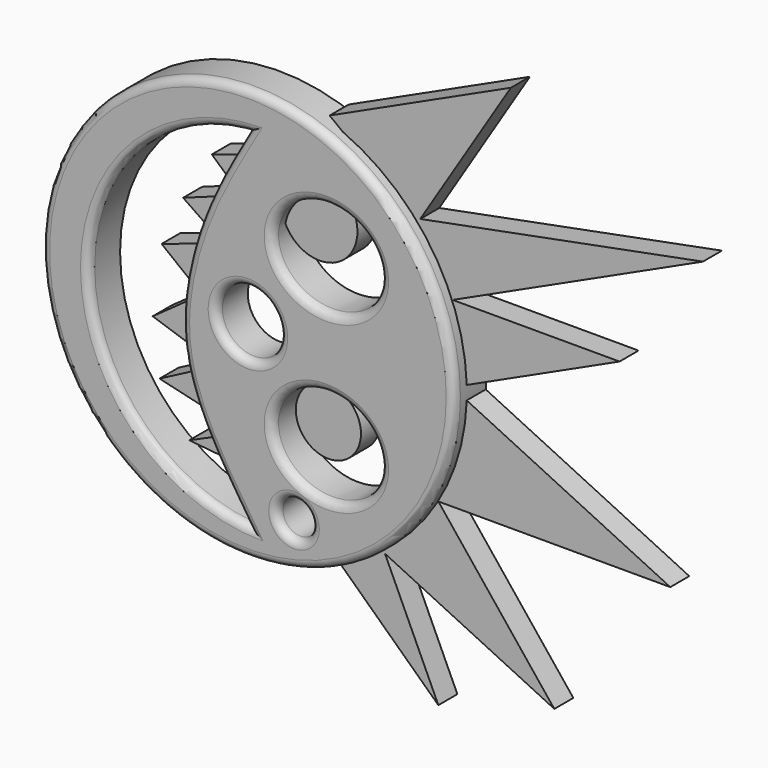
from build123d import *

# Parameters (mm, degrees)
F0_R     = 26.0210777057
F1_DEPTH = 5
F2_R     = 4.0159467608
F2_R_2   = 2.1900892751
F3_DEPTH = 5.0038
F4_R     = 4.7816675569
F5_DEPTH = 3
F4_R_2   = 4.1098377278
F6_R     = 1


# Not quite as in the source:
# - a feature names something its author has since deleted; it is built from what else it names


with BuildPart() as f1:
    # F0 (on Front) → F1 (new body)
    with BuildSketch(Plane.XZ):
        Circle(F0_R)
    extrude(amount=F1_DEPTH)

    # F2 (on face) → F3 (cut)
    with BuildSketch(Plane(origin=(0, 0, 0), x_dir=(-1, 0, 0), z_dir=(0, 1, 0))):
        with BuildLine():
            add(Edge.make_bspline(
                [(-3.0610915273, 10.4437181726), (-3.0610915273, 20.7679885804), (-13.3247473277, 15.6058533765), (-23.5884031281, 10.4437181726), (-13.3247473277, 5.2815829687), (-3.0610915273, 0.1194477649), (-3.0610915273, 10.4437181726)],
                knots=[0, 0, 0, 2.0943951024, 2.0943951024, 4.1887902048, 4.1887902048, 6.2831853072, 6.2831853072, 6.2831853072], degree=2, weights=[1, 0.5, 1, 0.5, 1, 0.5, 1]))
        make_face()
        with BuildLine():
            add(Edge.make_bspline(
                [(-3.0610915273, -10.4437181726), (-3.0610915273, -0.1194477649), (-13.3247473277, -5.2815829687), (-23.5884031281, -10.4437181726), (-13.3247473277, -15.6058533765), (-3.0610915273, -20.7679885804), (-3.0610915273, -10.4437181726)],
                knots=[0, 0, 0, 2.0943951024, 2.0943951024, 4.1887902048, 4.1887902048, 6.2831853072, 6.2831853072, 6.2831853072], degree=2, weights=[1, 0.5, 1, 0.5, 1, 0.5, 1]))
        make_face()
        with BuildLine():
            add(Edge.make_bspline(
                [(0, 21.2571714073), (2.1395691334, 17.5349161848), (6.4343134883, 10.0632554868), (9.437117435, -3.3422966836), (5.9538411419, -13.4085659123), (2.0003803602, -19.410914793), (0, -22.4479958415)],
                knots=[0, 0, 0, 0, 0.2628002315, 0.5275173365, 0.7609322331, 1, 1, 1, 1], degree=3))
            ThreePointArc((0, -22.4479958415), (20.127904461, -0.5954122171), (0, 21.2571714073))
        make_face()
        Circle(F2_R)
        with Locations((-5.8165974915, -19.9184641242)):
            Circle(F2_R_2)
    extrude(amount=-F3_DEPTH, mode=Mode.SUBTRACT)

    # F4 (on Front) → F5 (join)
    with BuildSketch(Plane.XZ):
        Polygon((31.5703637898, 35.6537438929), (8.7103629485, 25.1381471753), (15.68903464, 19.7567166877), (17.6219893204, 9.7053471258), (20.1403633691, -3.3902047333), (10.0819636136, -24.2394600064), (22.4263649434, -35.8924969307), (15.68903464, -21.2461215951), (37.0567627251, -31.5546505153), (22.4263649434, -13.2666537538), (51.6871623695, -13.2666537538), (24.1877730575, 0), (45.2863611281, 9.7053471258), (24.240220058, 9.7053471258), (55.8019652963, 24.2237448692), (20.1403633691, 17.3657480627), align=None)
        Polygon((-2.4479390122, 12.6461079344), (0, 18.0115178227), (-6.1536575668, 15.9823913127), align=None)
        Polygon((0, -17.575038597), (-1.9107642584, -13.542169705), (-8.998112753, -16.6923217475), align=None)
        Polygon((-1.9107642584, -13.542169705), (-5.3198472597, -7.1840547025), (-12.7467457205, -11.0646346584), (-4.5189405791, -13.0063341931), align=None)
        Polygon((-5.3198472597, -7.1840547025), (-7.4151288718, 0), (-13.6155430228, -4.4230874628), align=None)
        Polygon((-7.4151288718, 0), (-4.7596772201, 6.5502687357), (-12.4914376065, 3.9838966914), align=None)
        Polygon((-4.7596772201, 6.5502687357), (-2.4479390122, 12.6461079344), (-9.7722588107, 9.9908988923), align=None)
        with Locations((7.4385679327, 13.3894300088)):
            Circle(F4_R)
    extrude(amount=F5_DEPTH)

    # F6
    f6_edges = [f1.edges().sort_by_distance(p)[0] for p in [
        (-26.021078, -5, 0),
        (16.745966, -5, -10.443718),
        (16.745966, -5, 10.443718),
        (-20.127904, -5, -0.595412),
        (-8.299689, -5, -0.738162),
        (8.006687, -5, -19.918464),
        (4.015947, -5, 0),
    ]]
    fillet(f6_edges, radius=F6_R)


with BuildPart() as f5:
    # F4 (on Front) → F5, piece 2 (new body)
    with BuildSketch(Plane.XZ):
        with Locations((8.55435431, -8.9262863621)):
            Circle(F4_R_2)
    extrude(amount=F5_DEPTH)


solid = Compound([f1.part, f5.part])
